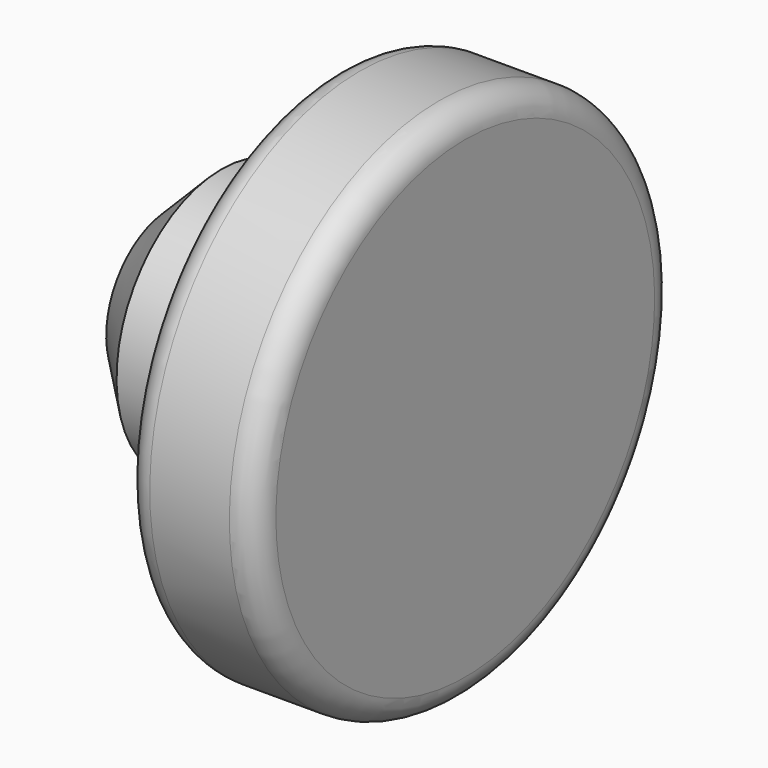
from build123d import *

# Parameters (mm, degrees)
F2_SIZE = 1
F3_R    = 0.5


with BuildPart() as f1:
    # F0 (on Front) → F1 (revolve)
    with BuildSketch(Plane.XZ):
        Polygon((0, 5.08), (0, 2.54), (-3.175, 2.54), (-3.175, 0), (2.54, 0), (2.54, 5.08), align=None)
    revolve(axis=Axis((-24.3718145439, 0, 0), (-1, 0, 0)))

    # F2
    f2_edges = [f1.edges().sort_by_distance(p)[0] for p in [
        (-3.175, 0, -2.54),
    ]]
    chamfer(f2_edges, length=F2_SIZE)

    # F3
    f3_edges = [f1.edges().sort_by_distance(p)[0] for p in [
        (0, 0, -5.08),
        (2.54, 0, -5.08),
    ]]
    fillet(f3_edges, radius=F3_R)


solid = f1.part
